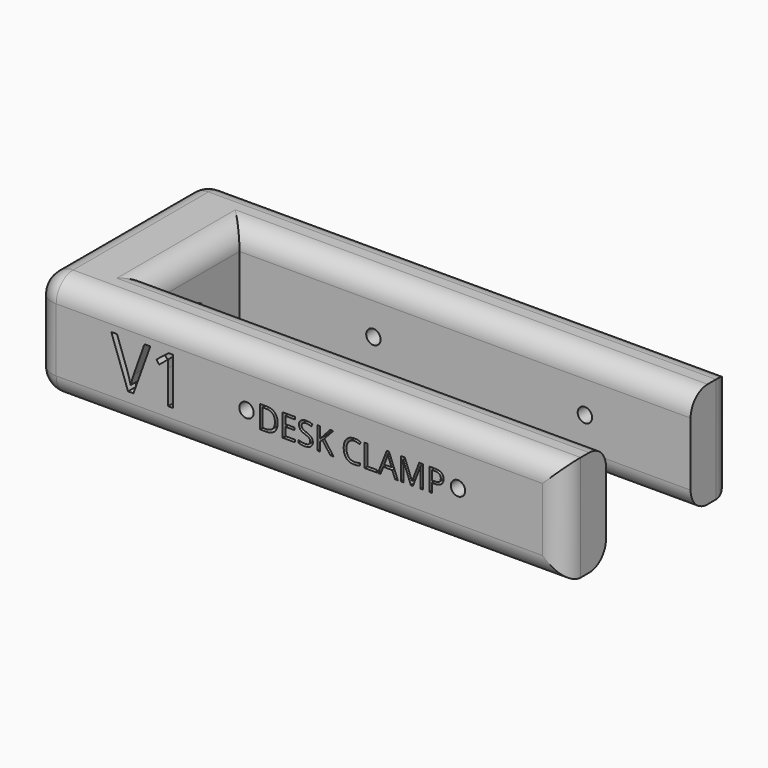
from build123d import *

# Parameters (mm, degrees)
F1_DEPTH       = 25.4
F3_D           = 3.4544
F5_D           = 3.4544
F6_D           = 3.4544
F7_TEXT_SIZE   = 7.5496138177
F7_TEXT_SIZE_2 = 15.7614723624
F8_DEPTH       = 2.54
F9_R           = 5.08


# Not quite as in the source:
# - Text() gives the source's letters only with a copy of the font that has no kerning and outlines rounded to 1/6400 em; it was checked with that copy


with BuildPart() as f1:
    # F0 (on Top) → F1 (new body)
    with BuildSketch(Plane.XY):
        Polygon((87.946691764, -8.7352859236), (-20.4159402835, -8.7352859236), (-20.4159402835, 16.6647140764), (87.946691764, 16.6647140764), (87.946691764, 29.3647140764), (-39.053308236, 29.3647140764), (-39.053308236, -21.4352859236), (87.946691764, -21.4352859236), align=None)
    extrude(amount=F1_DEPTH)

    # F3 (through all)
    with Locations(Plane.XZ.offset(21.4352859236)):
        with Locations((62.546691764, 12.7)):
            Hole(F3_D / 2)

    # F5 (through all)
    with Locations(Plane(origin=(-39.053308236, 0, 0), x_dir=(0, -1, 0), z_dir=(-1, 0, 0))):
        with Locations((-3.9647140764, 12.7)):
            Hole(F5_D / 2)

    # F6 (through all)
    with Locations(Plane.XZ.offset(21.4352859236)):
        with Locations((11.746691764, 12.7)):
            Hole(F6_D / 2)

    # F7 (on face) → F8 (cut)
    with BuildSketch(Plane.XZ.offset(21.4352859236)):
        with Locations((14.1878500581, 9.6845328808)):
            Text('DESK CLAMP', F7_TEXT_SIZE, font='Open Sans', text_align=(TextAlign.LEFT, TextAlign.BOTTOM))
        with Locations((-20.7490473986, 7.4221757241)):
            Text('V1', F7_TEXT_SIZE_2, font='Open Sans', text_align=(TextAlign.LEFT, TextAlign.BOTTOM))
    extrude(amount=-F8_DEPTH, mode=Mode.SUBTRACT)

    # F9
    f9_edges = [f1.edges().sort_by_distance(p)[0] for p in [
        (33.765376, -8.735286, 25.4),
        (-20.41594, 3.964714, 25.4),
        (33.765376, 16.664714, 25.4),
        (24.446692, 29.364714, 25.4),
        (-39.053308, 3.964714, 25.4),
        (24.446692, -21.435286, 0),
        (24.446692, 29.364714, 0),
        (-39.053308, 3.964714, 0),
        (24.446692, -21.435286, 25.4),
        (87.946692, -21.435286, 12.7),
        (-39.053308, 29.364714, 12.7),
        (-39.053308, -21.435286, 12.7),
        (33.765376, 16.664714, 0),
        (-20.41594, 3.964714, 0),
        (33.765376, -8.735286, 0),
        (87.946692, 29.364714, 12.7),
    ]]
    fillet(f9_edges, radius=F9_R)


solid = f1.part
